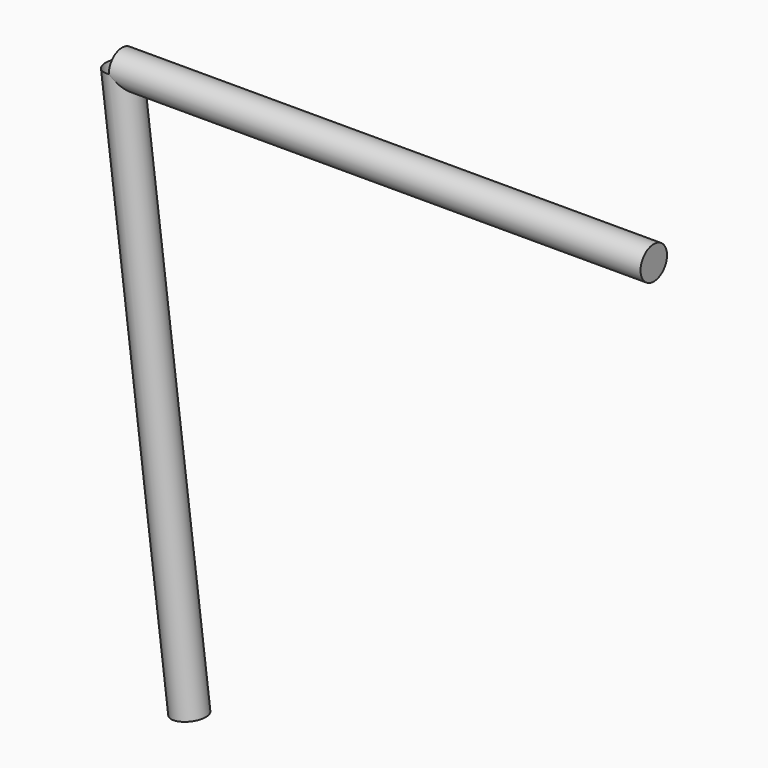
from build123d import *

# Parameters (mm, degrees)
F3_R = 16.5
F6_R = 16.5


# Not quite as in the source:
# - the program builds the solid bodies; features that only make, move or delete a surface that nothing else refers to are left out


with BuildPart() as f4:
    # F4: sweep along a path in F0
    with BuildLine(Plane.XZ) as f4_path:
        Line((0, 22.5), (-67.0281388728, 568.4003834027))
    # F3 (on line) → F4 (sweep)
    with BuildSketch(Plane(origin=(-69.7497601983, 0, 568.0662103233), x_dir=(0.9925461516, 0, 0.1218693434), z_dir=(-0.1218693434, 0, 0.9925461516))):
        with Locations((2.7420602266, 0)):
            Circle(F3_R)
    sweep(path=f4_path.line)

    # F7: sweep along a path in F0
    with BuildLine(Plane.XZ) as f7_path:
        Line((-67.0281388728, 568.4003834027), (462.9718611272, 568.4003834027))
    # F6 (on line) → F7 (sweep)
    with BuildSketch(Plane.YZ.offset(462.9718611272)):
        with Locations((0, 568.453848362)):
            Circle(F6_R)
    sweep(path=f7_path.line)


solid = f4.part
